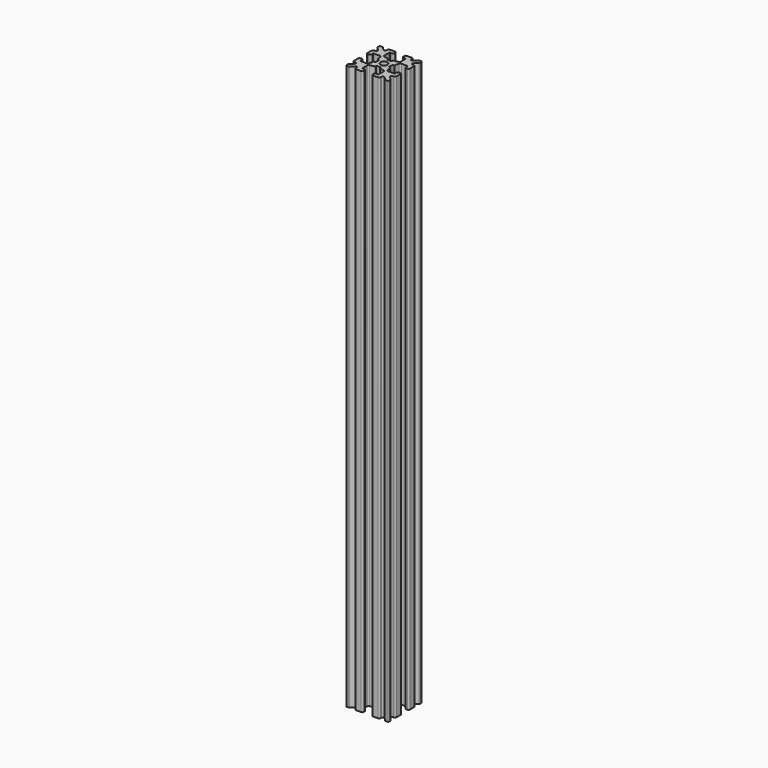
from build123d import *

# Parameters (mm, degrees)
F1_DEPTH = 200


# Not quite as in the source:
# - ends of sketch curves that miss each other by under 0.0002 mm in the source are joined


with BuildPart() as f1:
    # F0 (on Top) → F1 (new body)
    with BuildSketch(Plane.XY):
        with BuildLine():
            Line((-1.814515, 17.736209), (-2.91158, 17.736209))
            ThreePointArc((-2.91158, 17.736209), (-3.2776965235, 16.8523255235), (-4.16158, 16.486209))
            Line((-4.16158, 16.486209), (-4.16158, 15.389144))
            Line((-4.16158, 15.389144), (-3.53608, 15.389144))
            ThreePointArc((-3.53608, 15.389144), (-3.3946586438, 15.3305653562), (-3.33608, 15.189144))
            Line((-3.33608, 15.189144), (-3.33608, 14.961318))
            ThreePointArc((-3.33608, 14.961318), (-3.2922023866, 14.8363147984), (-3.1798219959, 14.7661600184))
            Line((-3.1798219959, 14.7661600184), (-1.652224, 14.423767))
            ThreePointArc((-1.652224, 14.423767), (-1.3712737286, 14.2483796232), (-1.26158, 13.935872))
            Line((-1.26158, 13.935872), (-1.26158, 11.836209))
            ThreePointArc((-1.26158, 11.836209), (-1.3201586438, 11.6947876438), (-1.46158, 11.636209))
            Line((-1.46158, 11.636209), (-2.06158, 11.636209))
            ThreePointArc((-2.06158, 11.636209), (-2.4151333906, 11.4897623906), (-2.56158, 11.136209))
            Line((-2.56158, 11.136209), (-2.56158, 10.736209))
            ThreePointArc((-2.56158, 10.736209), (-2.4151333906, 10.3826556094), (-2.06158, 10.236209))
            Line((-2.06158, 10.236209), (-0.26158, 10.236209))
            ThreePointArc((-0.26158, 10.236209), (0.0919733906, 10.3826556094), (0.23842, 10.736209))
            Line((0.23842, 10.736209), (0.23842, 11.068442))
            ThreePointArc((0.23842, 11.068442), (0.5470786105, 11.5303819016), (1.0919738906, 11.4219948906))
            Line((1.0919738906, 11.4219948906), (2.131313, 10.382656))
            ThreePointArc((2.131313, 10.382656), (2.2935249572, 10.274269369), (2.484867, 10.236209))
            Line((2.484867, 10.236209), (3.08842, 10.236209))
            ThreePointArc((3.08842, 10.236209), (3.2651966953, 10.3094323047), (3.33842, 10.486209))
            Line((3.33842, 10.486209), (3.33842, 11.089762))
            ThreePointArc((3.33842, 11.089762), (3.3003597663, 11.2811037162), (3.1919733906, 11.4433153906))
            Line((3.1919733906, 11.4433153906), (2.152634, 12.482656))
            ThreePointArc((2.152634, 12.482656), (2.0442472337, 13.0275507162), (2.506187, 13.336209))
            Line((2.506187, 13.336209), (2.83842, 13.336209))
            ThreePointArc((2.83842, 13.336209), (3.1919733906, 13.4826556094), (3.33842, 13.836209))
            Line((3.33842, 13.836209), (3.33842, 15.636209))
            ThreePointArc((3.33842, 15.636209), (3.1919733906, 15.9897623906), (2.83842, 16.136209))
            Line((2.83842, 16.136209), (2.43842, 16.136209))
            ThreePointArc((2.43842, 16.136209), (2.0848666094, 15.9897623906), (1.93842, 15.636209))
            Line((1.93842, 15.636209), (1.93842, 15.036209))
            ThreePointArc((1.93842, 15.036209), (1.8798413562, 14.8947876438), (1.73842, 14.836209))
            Line((1.73842, 14.836209), (-0.361243, 14.836209))
            ThreePointArc((-0.361243, 14.836209), (-0.6737506232, 14.9459027286), (-0.8491377407, 15.2268530581))
            Line((-0.8491377407, 15.2268530581), (-1.191531, 16.754451))
            ThreePointArc((-1.191531, 16.754451), (-1.2616857984, 16.8668313866), (-1.386689, 16.910709))
            Line((-1.386689, 16.910709), (-1.614515, 16.910709))
            ThreePointArc((-1.614515, 16.910709), (-1.7559363562, 16.9692876438), (-1.814515, 17.110709))
            Line((-1.814515, 17.110709), (-1.814515, 17.736209))
        make_face()
        with BuildLine():
            ThreePointArc((-4.16158, 18.986209), (-3.2776965235, 18.6200924765), (-2.91158, 17.736209))
            Line((-2.91158, 17.736209), (-1.814515, 17.736209))
            Line((-1.814515, 17.736209), (-1.814515, 18.361709))
            ThreePointArc((-1.814515, 18.361709), (-1.7559363562, 18.5031303562), (-1.614515, 18.561709))
            Line((-1.614515, 18.561709), (-1.386689, 18.561709))
            ThreePointArc((-1.386689, 18.561709), (-1.2616857984, 18.6055866134), (-1.1915310184, 18.7179670041))
            Line((-1.1915310184, 18.7179670041), (-0.849138, 20.245565))
            ThreePointArc((-0.849138, 20.245565), (-0.6737506232, 20.5265152714), (-0.361243, 20.636209))
            Line((-0.361243, 20.636209), (1.73842, 20.636209))
            ThreePointArc((1.73842, 20.636209), (1.8798413562, 20.5776303562), (1.93842, 20.436209))
            Line((1.93842, 20.436209), (1.93842, 19.836209))
            ThreePointArc((1.93842, 19.836209), (2.0848666094, 19.4826556094), (2.43842, 19.336209))
            Line((2.43842, 19.336209), (2.83842, 19.336209))
            ThreePointArc((2.83842, 19.336209), (3.1919733906, 19.4826556094), (3.33842, 19.836209))
            Line((3.33842, 19.836209), (3.33842, 21.636209))
            ThreePointArc((3.33842, 21.636209), (3.1919733906, 21.9897623906), (2.83842, 22.136209))
            Line((2.83842, 22.136209), (2.506187, 22.136209))
            ThreePointArc((2.506187, 22.136209), (2.0442472337, 22.4448672838), (2.1526336094, 22.9897623906))
            Line((2.1526336094, 22.9897623906), (3.191974, 24.029102))
            ThreePointArc((3.191974, 24.029102), (3.3003597663, 24.1913142838), (3.33842, 24.382656))
            Line((3.33842, 24.382656), (3.33842, 24.986209))
            ThreePointArc((3.33842, 24.986209), (3.2651966953, 25.1629856953), (3.08842, 25.236209))
            Line((3.08842, 25.236209), (2.484867, 25.236209))
            ThreePointArc((2.484867, 25.236209), (2.2935249572, 25.198148631), (2.1313131094, 25.0897618906))
            Line((2.1313131094, 25.0897618906), (1.091974, 24.050423))
            ThreePointArc((1.091974, 24.050423), (0.5470786105, 23.9420360984), (0.23842, 24.403976))
            Line((0.23842, 24.403976), (0.23842, 24.736209))
            ThreePointArc((0.23842, 24.736209), (0.0919733906, 25.0897623906), (-0.26158, 25.236209))
            Line((-0.26158, 25.236209), (-2.06158, 25.236209))
            ThreePointArc((-2.06158, 25.236209), (-2.4151333906, 25.0897623906), (-2.56158, 24.736209))
            Line((-2.56158, 24.736209), (-2.56158, 24.336209))
            ThreePointArc((-2.56158, 24.336209), (-2.4151333906, 23.9826556094), (-2.06158, 23.836209))
            Line((-2.06158, 23.836209), (-1.46158, 23.836209))
            ThreePointArc((-1.46158, 23.836209), (-1.3201586438, 23.7776303562), (-1.26158, 23.636209))
            Line((-1.26158, 23.636209), (-1.26158, 21.536546))
            ThreePointArc((-1.26158, 21.536546), (-1.3712737286, 21.2240383768), (-1.6522240581, 21.0486512593))
            Line((-1.6522240581, 21.0486512593), (-3.179822, 20.706258))
            ThreePointArc((-3.179822, 20.706258), (-3.2922023866, 20.6361032016), (-3.33608, 20.5111))
            Line((-3.33608, 20.5111), (-3.33608, 20.283274))
            ThreePointArc((-3.33608, 20.283274), (-3.3946586438, 20.1418526438), (-3.53608, 20.083274))
            Line((-3.53608, 20.083274), (-4.16158, 20.083274))
            Line((-4.16158, 20.083274), (-4.16158, 18.986209))
        make_face()
        with BuildLine():
            ThreePointArc((-5.41158, 17.736209), (-5.0454634765, 18.6200924765), (-4.16158, 18.986209))
            Line((-4.16158, 18.986209), (-4.16158, 20.083274))
            Line((-4.16158, 20.083274), (-4.78708, 20.083274))
            ThreePointArc((-4.78708, 20.083274), (-4.9285013562, 20.1418526438), (-4.98708, 20.283274))
            Line((-4.98708, 20.283274), (-4.98708, 20.5111))
            ThreePointArc((-4.98708, 20.5111), (-5.0309576134, 20.6361032016), (-5.1433380041, 20.7062579816))
            Line((-5.1433380041, 20.7062579816), (-6.670936, 21.048651))
            ThreePointArc((-6.670936, 21.048651), (-6.9518862714, 21.2240383768), (-7.06158, 21.536546))
            Line((-7.06158, 21.536546), (-7.06158, 23.636209))
            ThreePointArc((-7.06158, 23.636209), (-7.0030013562, 23.7776303562), (-6.86158, 23.836209))
            Line((-6.86158, 23.836209), (-6.26158, 23.836209))
            ThreePointArc((-6.26158, 23.836209), (-5.9080266094, 23.9826556094), (-5.76158, 24.336209))
            Line((-5.76158, 24.336209), (-5.76158, 24.736209))
            ThreePointArc((-5.76158, 24.736209), (-5.9080266094, 25.0897623906), (-6.26158, 25.236209))
            Line((-6.26158, 25.236209), (-8.06158, 25.236209))
            ThreePointArc((-8.06158, 25.236209), (-8.4151333906, 25.0897623906), (-8.56158, 24.736209))
            Line((-8.56158, 24.736209), (-8.56158, 24.403976))
            ThreePointArc((-8.56158, 24.403976), (-8.8702382838, 23.9420362337), (-9.4151333906, 24.0504226094))
            Line((-9.4151333906, 24.0504226094), (-10.454473, 25.089762))
            ThreePointArc((-10.454473, 25.089762), (-10.6166842838, 25.1981487663), (-10.808026, 25.236209))
            Line((-10.808026, 25.236209), (-11.41158, 25.236209))
            ThreePointArc((-11.41158, 25.236209), (-11.5883566953, 25.1629856953), (-11.66158, 24.986209))
            Line((-11.66158, 24.986209), (-11.66158, 24.382656))
            ThreePointArc((-11.66158, 24.382656), (-11.623519631, 24.1913139572), (-11.5151328906, 24.0291021094))
            Line((-11.5151328906, 24.0291021094), (-10.475793, 22.989762))
            ThreePointArc((-10.475793, 22.989762), (-10.367407369, 22.4448669572), (-10.829347, 22.136209))
            Line((-10.829347, 22.136209), (-11.16158, 22.136209))
            ThreePointArc((-11.16158, 22.136209), (-11.5151333906, 21.9897623906), (-11.66158, 21.636209))
            Line((-11.66158, 21.636209), (-11.66158, 19.836209))
            ThreePointArc((-11.66158, 19.836209), (-11.5151333906, 19.4826556094), (-11.16158, 19.336209))
            Line((-11.16158, 19.336209), (-10.76158, 19.336209))
            ThreePointArc((-10.76158, 19.336209), (-10.4080266094, 19.4826556094), (-10.26158, 19.836209))
            Line((-10.26158, 19.836209), (-10.26158, 20.436209))
            ThreePointArc((-10.26158, 20.436209), (-10.2030013562, 20.5776303562), (-10.06158, 20.636209))
            Line((-10.06158, 20.636209), (-7.961916, 20.636209))
            ThreePointArc((-7.961916, 20.636209), (-7.6494084622, 20.5265153397), (-7.4740213072, 20.2455651553))
            Line((-7.4740213072, 20.2455651553), (-7.131629, 18.717967))
            ThreePointArc((-7.131629, 18.717967), (-7.0614742016, 18.6055866134), (-6.936471, 18.561709))
            Line((-6.936471, 18.561709), (-6.708644, 18.561709))
            ThreePointArc((-6.708644, 18.561709), (-6.5672226438, 18.5031303562), (-6.508644, 18.361709))
            Line((-6.508644, 18.361709), (-6.508644, 17.736209))
            Line((-6.508644, 17.736209), (-5.41158, 17.736209))
        make_face()
        with BuildLine():
            Line((-4.16158, 15.389144), (-4.16158, 16.486209))
            ThreePointArc((-4.16158, 16.486209), (-5.0454634765, 16.8523255235), (-5.41158, 17.736209))
            Line((-5.41158, 17.736209), (-6.508644, 17.736209))
            Line((-6.508644, 17.736209), (-6.508644, 17.110709))
            ThreePointArc((-6.508644, 17.110709), (-6.5672226438, 16.9692876438), (-6.708644, 16.910709))
            Line((-6.708644, 16.910709), (-6.936471, 16.910709))
            ThreePointArc((-6.936471, 16.910709), (-7.0614742016, 16.8668313866), (-7.1316289816, 16.7544509959))
            Line((-7.1316289816, 16.7544509959), (-7.474022, 15.226853))
            ThreePointArc((-7.474022, 15.226853), (-7.6494084622, 14.9459026603), (-7.961916, 14.836209))
            Line((-7.961916, 14.836209), (-10.06158, 14.836209))
            ThreePointArc((-10.06158, 14.836209), (-10.2030013562, 14.8947876438), (-10.26158, 15.036209))
            Line((-10.26158, 15.036209), (-10.26158, 15.636209))
            ThreePointArc((-10.26158, 15.636209), (-10.4080266094, 15.9897623906), (-10.76158, 16.136209))
            Line((-10.76158, 16.136209), (-11.16158, 16.136209))
            ThreePointArc((-11.16158, 16.136209), (-11.5151333906, 15.9897623906), (-11.66158, 15.636209))
            Line((-11.66158, 15.636209), (-11.66158, 13.836209))
            ThreePointArc((-11.66158, 13.836209), (-11.5151333906, 13.4826556094), (-11.16158, 13.336209))
            Line((-11.16158, 13.336209), (-10.829347, 13.336209))
            ThreePointArc((-10.829347, 13.336209), (-10.367407369, 13.0275510428), (-10.4757931094, 12.4826561094))
            Line((-10.4757931094, 12.4826561094), (-11.515133, 11.443316))
            ThreePointArc((-11.515133, 11.443316), (-11.623519631, 11.2811040428), (-11.66158, 11.089762))
            Line((-11.66158, 11.089762), (-11.66158, 10.486209))
            ThreePointArc((-11.66158, 10.486209), (-11.5883566953, 10.3094323047), (-11.41158, 10.236209))
            Line((-11.41158, 10.236209), (-10.808026, 10.236209))
            ThreePointArc((-10.808026, 10.236209), (-10.6166842838, 10.2742692337), (-10.4544726094, 10.3826556094))
            Line((-10.4544726094, 10.3826556094), (-9.415133, 11.421995))
            ThreePointArc((-9.415133, 11.421995), (-8.8702382838, 11.5303817663), (-8.56158, 11.068442))
            Line((-8.56158, 11.068442), (-8.56158, 10.736209))
            ThreePointArc((-8.56158, 10.736209), (-8.4151333906, 10.3826556094), (-8.06158, 10.236209))
            Line((-8.06158, 10.236209), (-6.26158, 10.236209))
            ThreePointArc((-6.26158, 10.236209), (-5.9080266094, 10.3826556094), (-5.76158, 10.736209))
            Line((-5.76158, 10.736209), (-5.76158, 11.136209))
            ThreePointArc((-5.76158, 11.136209), (-5.9080266094, 11.4897623906), (-6.26158, 11.636209))
            Line((-6.26158, 11.636209), (-6.86158, 11.636209))
            ThreePointArc((-6.86158, 11.636209), (-7.0030013562, 11.6947876438), (-7.06158, 11.836209))
            Line((-7.06158, 11.836209), (-7.06158, 13.935872))
            ThreePointArc((-7.06158, 13.935872), (-6.9518862714, 14.2483796232), (-6.6709359419, 14.4237667407))
            Line((-6.6709359419, 14.4237667407), (-5.143338, 14.76616))
            ThreePointArc((-5.143338, 14.76616), (-5.0309576134, 14.8363147984), (-4.98708, 14.961318))
            Line((-4.98708, 14.961318), (-4.98708, 15.189144))
            ThreePointArc((-4.98708, 15.189144), (-4.9285013562, 15.3305653562), (-4.78708, 15.389144))
            Line((-4.78708, 15.389144), (-4.16158, 15.389144))
        make_face()
    extrude(amount=F1_DEPTH)


solid = f1.part
